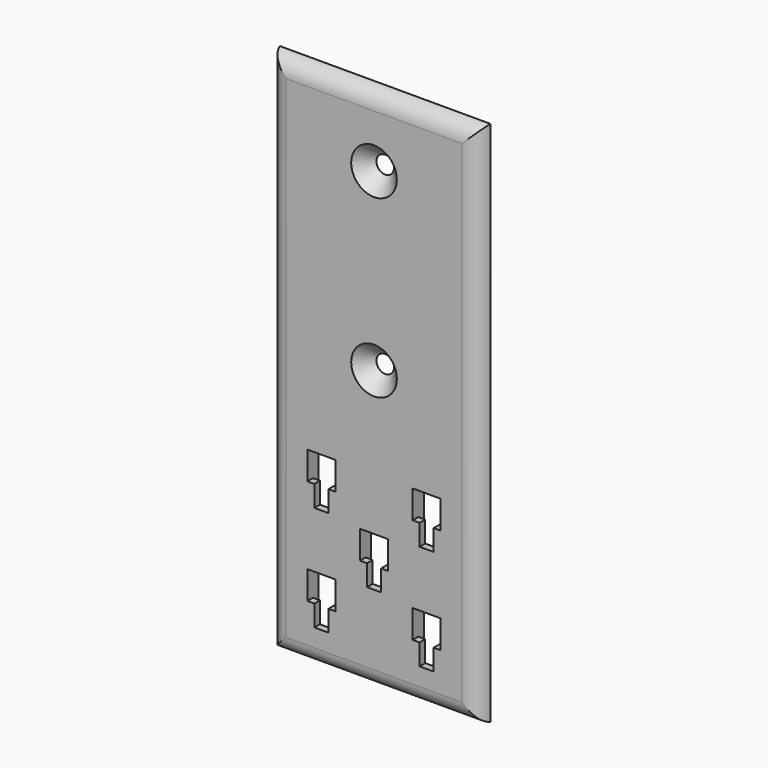
from build123d import *
from build123d import SkipClean  # not in build123d's __all__

# Parameters (mm, degrees)
F0_R        = 1.5
F1_DEPTH    = 2
F0_W        = 2
F0_H        = 6
F0_H_2      = 2
F0_W_2      = 4
F2_DEPTH    = 2
F4_T1_DEPTH = 84.4948974279
F4_T3_DEPTH = 174.4948974279


# Not quite as in the source:
# - a fillet or chamfer that OpenCascade refuses, or shapes differently, is made with other operations: its cross-section is extruded or revolved along the edge and cut away or added


with BuildPart() as f1:
    # F0 (on Front) → F1 (new body)
    with BuildSketch(Plane.XZ):
        with BuildLine():
            Line((-30, 150), (-30, 80))
            Line((-30, 80), (-1.5, 80))
            ThreePointArc((-1.5, 80), (0, 81.5), (1.5, 80))
            Line((1.5, 80), (30, 80))
            Line((30, 80), (30, 150))
            Line((30, 150), (-30, 150))
        make_face()
        with Locations((0, 130)):
            Circle(F0_R, mode=Mode.SUBTRACT)
        with BuildLine():
            Line((-30, 0), (0, 0))
            Line((0, 0), (30, 0))
            Line((30, 0), (30, 80))
            Line((30, 80), (1.5, 80))
            ThreePointArc((1.5, 80), (0, 78.5), (-1.5, 80))
            Line((-1.5, 80), (-30, 80))
            Line((-30, 80), (-30, 0))
        make_face()
        Polygon((-11, 24), (-11, 16), (-11, 10), (-11, 8), (-13, 8), (-17, 8), (-19, 8), (-19, 10), (-19, 16), (-19, 24), align=None, mode=Mode.SUBTRACT)
        Polygon((-11, 48), (-11, 46), (-11, 40), (-11, 38), (-13, 38), (-17, 38), (-19, 38), (-19, 40), (-19, 46), (-19, 48), (-19, 54), (-11, 54), align=None, mode=Mode.SUBTRACT)
        Polygon((4, 39), (4, 31), (4, 25), (4, 23), (2, 23), (-2, 23), (-4, 23), (-4, 25), (-4, 31), (-4, 39), align=None, mode=Mode.SUBTRACT)
        Polygon((19, 24), (19, 16), (19, 10), (19, 8), (17, 8), (13, 8), (11, 8), (11, 10), (11, 16), (11, 24), align=None, mode=Mode.SUBTRACT)
        Polygon((19, 54), (19, 46), (19, 40), (19, 38), (17, 38), (13, 38), (11, 38), (11, 40), (11, 46), (11, 54), align=None, mode=Mode.SUBTRACT)
    extrude(amount=-F1_DEPTH)

    # F0 (on Front) → F2 (join)
    with BuildSketch(Plane.XZ):
        with BuildLine():
            Line((-30, 0), (0, 0))
            Line((0, 0), (30, 0))
            Line((30, 0), (30, 80))
            Line((30, 80), (1.5, 80))
            ThreePointArc((1.5, 80), (0, 78.5), (-1.5, 80))
            Line((-1.5, 80), (-30, 80))
            Line((-30, 80), (-30, 0))
        make_face()
        Polygon((-11, 24), (-11, 16), (-11, 10), (-11, 8), (-13, 8), (-17, 8), (-19, 8), (-19, 10), (-19, 16), (-19, 24), align=None, mode=Mode.SUBTRACT)
        Polygon((-11, 48), (-11, 46), (-11, 40), (-11, 38), (-13, 38), (-17, 38), (-19, 38), (-19, 40), (-19, 46), (-19, 48), (-19, 54), (-11, 54), align=None, mode=Mode.SUBTRACT)
        Polygon((4, 39), (4, 31), (4, 25), (4, 23), (2, 23), (-2, 23), (-4, 23), (-4, 25), (-4, 31), (-4, 39), align=None, mode=Mode.SUBTRACT)
        Polygon((19, 24), (19, 16), (19, 10), (19, 8), (17, 8), (13, 8), (11, 8), (11, 10), (11, 16), (11, 24), align=None, mode=Mode.SUBTRACT)
        Polygon((19, 54), (19, 46), (19, 40), (19, 38), (17, 38), (13, 38), (11, 38), (11, 40), (11, 46), (11, 54), align=None, mode=Mode.SUBTRACT)
        with BuildLine():
            Line((-30, 150), (-30, 80))
            Line((-30, 80), (-1.5, 80))
            ThreePointArc((-1.5, 80), (0, 81.5), (1.5, 80))
            Line((1.5, 80), (30, 80))
            Line((30, 80), (30, 150))
            Line((30, 150), (-30, 150))
        make_face()
        with Locations((0, 130)):
            Circle(F0_R, mode=Mode.SUBTRACT)
        with Locations((-12, 43)):
            Rectangle(F0_W, F0_H)
        with Locations((-12, 39)):
            Rectangle(F0_W, F0_H_2)
        with Locations((-18, 43)):
            Rectangle(F0_W, F0_H)
        with Locations((-15, 39)):
            Rectangle(F0_W_2, F0_H_2)
        with Locations((-18, 39)):
            Rectangle(F0_W, F0_H_2)
        with Locations((18, 43)):
            Rectangle(F0_W, F0_H)
        with Locations((18, 39)):
            Rectangle(F0_W, F0_H_2)
        with Locations((12, 43)):
            Rectangle(F0_W, F0_H)
        with Locations((15, 39)):
            Rectangle(F0_W_2, F0_H_2)
        with Locations((12, 39)):
            Rectangle(F0_W, F0_H_2)
        with Locations((3, 28)):
            Rectangle(F0_W, F0_H)
        with Locations((3, 24)):
            Rectangle(F0_W, F0_H_2)
        with Locations((-3, 28)):
            Rectangle(F0_W, F0_H)
        with Locations((0, 24)):
            Rectangle(F0_W_2, F0_H_2)
        with Locations((-3, 24)):
            Rectangle(F0_W, F0_H_2)
        with Locations((-12, 13)):
            Rectangle(F0_W, F0_H)
        with Locations((-12, 9)):
            Rectangle(F0_W, F0_H_2)
        with Locations((-18, 13)):
            Rectangle(F0_W, F0_H)
        with Locations((-15, 9)):
            Rectangle(F0_W_2, F0_H_2)
        with Locations((-18, 9)):
            Rectangle(F0_W, F0_H_2)
        with Locations((18, 13)):
            Rectangle(F0_W, F0_H)
        with Locations((18, 9)):
            Rectangle(F0_W, F0_H_2)
        with Locations((12, 13)):
            Rectangle(F0_W, F0_H)
        with Locations((15, 9)):
            Rectangle(F0_W_2, F0_H_2)
        with Locations((12, 9)):
            Rectangle(F0_W, F0_H_2)
    with SkipClean():  # cleaning this boolean's faces spoils the solid; the shape is the same uncleaned
        extrude(amount=F2_DEPTH)

    # F3: chamfer of 5 on 2 edges, made by hand

    # F3_s1 → F3_t2 (revolve, cut)
    with BuildSketch(Plane.XY.offset(130)):
        Polygon((6.5, -2), (1.5, 3), (1.5, -2), align=None)
    revolve(axis=Axis((0, -2, 130), (0, -1, 0)), mode=Mode.SUBTRACT)

    # F3_s3 → F3_t4 (revolve, cut)
    with BuildSketch(Plane.XY.offset(80)):
        Polygon((-6.5, -2), (-1.5, 3), (-1.5, -2), align=None)
    revolve(axis=Axis((0, -2, 80), (0, 1, 0)), mode=Mode.SUBTRACT)

    # F4: fillet of radius 5 on 4 edges, made by hand

    # F4_s2 → F4_t1 (cut)
    with BuildSketch(Plane.YZ.offset(-42.2474487139)):
        with BuildLine():
            ThreePointArc((2, 0), (-0.8729833462, 1.7367018254), (-2, 4.8989794856))
            Line((-2, 4.8989794856), (-2, 0))
            Line((-2, 0), (2, 0))
        make_face()
        with BuildLine():
            ThreePointArc((-2, 145.1010205144), (-0.8729833462, 148.2632981746), (2, 150))
            Line((2, 150), (-2, 150))
            Line((-2, 150), (-2, 145.1010205144))
        make_face()
    extrude(amount=F4_T1_DEPTH, mode=Mode.SUBTRACT)

    # F4_s4 → F4_t3 (cut)
    with BuildSketch(Plane.XY.offset(-12.2474487139)):
        with BuildLine():
            ThreePointArc((-30, 2), (-28.2632981746, -0.8729833462), (-25.1010205144, -2))
            Line((-25.1010205144, -2), (-30, -2))
            Line((-30, -2), (-30, 2))
        make_face()
        with BuildLine():
            ThreePointArc((25.1010205144, -2), (28.2632981746, -0.8729833462), (30, 2))
            Line((30, 2), (30, -2))
            Line((30, -2), (25.1010205144, -2))
        make_face()
    extrude(amount=F4_T3_DEPTH, mode=Mode.SUBTRACT)


solid = f1.part
